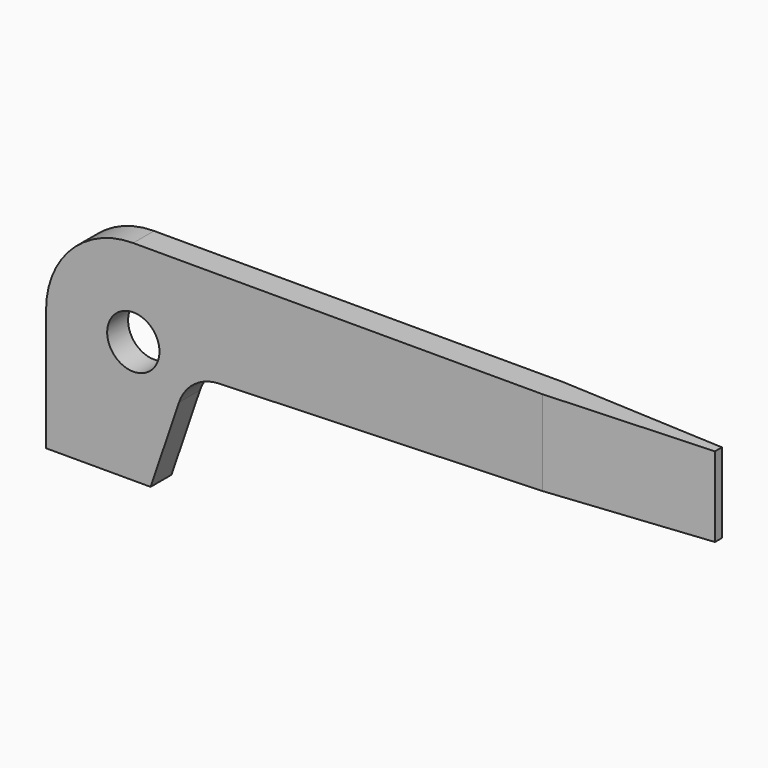
from build123d import *

# Parameters (mm, degrees)
F1_DEPTH = 2.38125
F2_R     = 2.38125
F3_DEPTH = 25.4
F5_DEPTH = 25.4


# Not quite as in the source:
# - a length typed as a fraction of an inch, garbled in the dataset ("3 / 203.2 mm" for 3/8 in), is restored


with BuildPart() as f1:
    # F0 (on Front) → F1 (new body)
    with BuildSketch(Plane.XZ):
        with BuildLine():
            Line((60.325, 19.05), (7.9375, 19.05))
            ThreePointArc((7.9375, 19.05), (2.3248399243, 16.7251600757), (0, 11.1125))
            Line((0, 11.1125), (0, 0))
            Line((0, 0), (9.525, 0))
            Line((9.525, 0), (12.1173647876, 7.6271664624))
            ThreePointArc((12.1173647876, 7.6271664624), (13.511585403, 9.5382986066), (15.7455205062, 10.3166373193))
            Line((15.7455205062, 10.3166373193), (60.325, 11.7718065158))
            Line((60.325, 11.7718065158), (60.325, 19.05))
        make_face()
    extrude(amount=F1_DEPTH)

    # F2 (on face) → F3 (cut)
    with BuildSketch(Plane.XZ.offset(2.38125)):
        with Locations((7.9502, 11.1125)):
            Circle(F2_R)
    extrude(amount=-F3_DEPTH, mode=Mode.SUBTRACT)

    # F4 (on face) → F5 (cut)
    with BuildSketch(Plane.XY.offset(19.05)):
        Polygon((45.24375, 0), (60.325, -0.79375), (60.325, 0), align=None)
        Polygon((60.325, -2.38125), (60.325, -1.5875), (45.24375, -2.38125), align=None)
    extrude(amount=-F5_DEPTH, mode=Mode.SUBTRACT)


solid = f1.part
